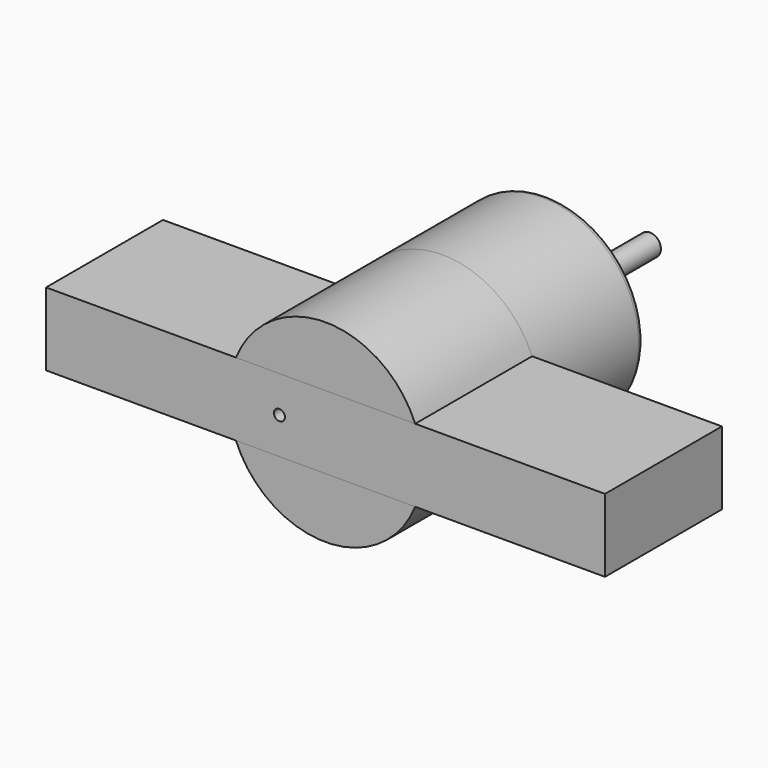
from build123d import *

# Parameters (mm, degrees)
F2_R     = 3
F4_DEPTH = 20
F5_DEPTH = 20
F6_R     = 1.5
F7_DEPTH = 1.5
F8_R     = 0.75
F9_DEPTH = 55.5010001


with BuildPart() as f1:
    # F0 (on Top) → F1 (revolve)
    with BuildSketch(Plane.XY):
        with BuildLine():
            Line((-13.25, 0), (0, 0))
            Line((0, 0), (0, 37))
            Line((0, 37), (-1.5, 37))
            Line((-1.5, 37), (-1.5, 16.6235913226))
            ThreePointArc((-1.5, 16.6235913226), (-6.4401709177, 12.3947665973), (-11.3803418353, 16.6235913226))
            Line((-11.3803418353, 16.6235913226), (-11.4607692348, 17.1388115494))
            ThreePointArc((-11.4607692348, 17.1388115494), (-12.4196143352, 17.8973036522), (-13.25, 17))
            Line((-13.25, 17), (-13.25, 0))
        make_face()
    revolve(axis=Axis((0, 18.5, 0), (0, -1, 0)))

    # F2
    f2_edges = [f1.edges().sort_by_distance(p)[0] for p in [
        (1.5, 16.623591, 0),
    ]]
    fillet(f2_edges, radius=F2_R)

    # F3 (on face) → F4 (join)
    with BuildSketch(Plane.XZ):
        with BuildLine():
            Line((-12.2703911918, 5), (-38.25, 5))
            Line((-38.25, 5), (-38.25, -5))
            Line((-38.25, -5), (-12.2703911918, -5))
            ThreePointArc((-12.2703911918, -5), (-13.25, 0), (-12.2703911918, 5))
        make_face()
        with BuildLine():
            Line((12.2703911918, 5), (-12.2703911918, 5))
            ThreePointArc((-12.2703911918, 5), (-13.25, 0), (-12.2703911918, -5))
            Line((-12.2703911918, -5), (12.2703911918, -5))
            ThreePointArc((12.2703911918, -5), (13.0027916866, -2.5475298535), (13.25, 0))
            ThreePointArc((13.25, 0), (13.0027916866, 2.5475298535), (12.2703911918, 5))
        make_face()
        with BuildLine():
            Line((38.25, 5), (12.2703911918, 5))
            ThreePointArc((12.2703911918, 5), (13.0027916866, 2.5475298535), (13.25, 0))
            ThreePointArc((13.25, 0), (13.0027916866, -2.5475298535), (12.2703911918, -5))
            Line((12.2703911918, -5), (38.25, -5))
            Line((38.25, -5), (38.25, 5))
        make_face()
    extrude(amount=F4_DEPTH)

    # F5 (add): faces of the model
    f5_faces = [f1.faces().sort_by_distance(p)[0] for p in [
        (0, 0, 8.4077666552),
        (0, 0, -8.4077666552),
    ]]
    extrude(f5_faces, amount=F5_DEPTH)

    # F6 (on face) → F7 (cut)
    with BuildSketch(Plane(origin=(0, 37, 0), x_dir=(-1, 0, 0), z_dir=(0, 1, 0))):
        Circle(F6_R)
    extrude(amount=-F7_DEPTH, mode=Mode.SUBTRACT)

    # F8 (on face) → F9 (cut, through all)
    with BuildSketch(Plane.XZ.offset(20)):
        with Locations((-6.3117844984, 0)):
            Circle(F8_R)
    extrude(amount=-F9_DEPTH, mode=Mode.SUBTRACT)


solid = f1.part
